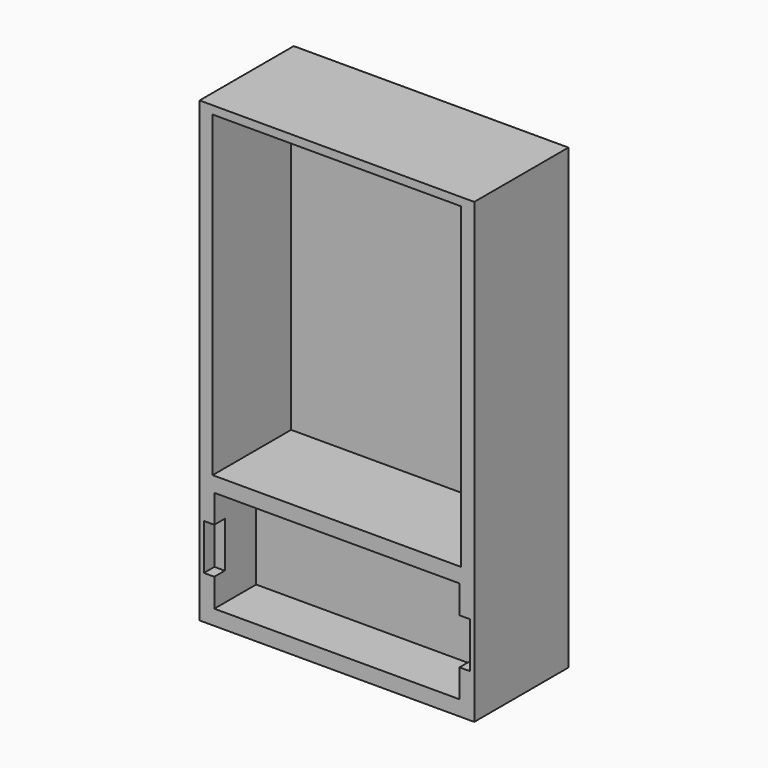
from build123d import *

# Parameters (mm, degrees)
F0_W     = 21
F0_H     = 35
F0_W_2   = 19
F0_H_2   = 24.2712582345
F1_DEPTH = 9
F2_DEPTH = 1.5
F3_DEPTH = 5
F0_W_3   = 0.7944880121
F0_H_3   = 3.5
F4_DEPTH = 8


# Not quite as in the source:
# - a feature names something its author has since deleted; it is built from what else it names


with BuildPart() as f1:
    # F0 (on Front) → F1 (new body)
    with BuildSketch(Plane.XZ):
        Rectangle(F0_W, F0_H)
        Polygon((-9.3731830162, -10.6923110513), (-9.3731830162, -8.5423110513), (9.3731830162, -8.5423110513), (9.3731830162, -10.6923110513), (10.1676710284, -10.6923110513), (10.1676710284, -14.1923110513), (9.3731830162, -14.1923110513), (9.3731830162, -16.3423110513), (-9.3731830162, -16.3423110513), (-9.3731830162, -14.1923110513), (-10.1676710284, -14.1923110513), (-10.1676710284, -10.6923110513), align=None, mode=Mode.SUBTRACT)
        with Locations((0, 4.7412435117)):
            Rectangle(F0_W_2, F0_H_2, mode=Mode.SUBTRACT)
    extrude(amount=F1_DEPTH)

    # F0 (on Front) → F2 (join)
    with BuildSketch(Plane.XZ):
        with Locations((0, 4.7412435117)):
            Rectangle(F0_W_2, F0_H_2)
    extrude(amount=F2_DEPTH)

    # F0 (on Front) → F3 (join)
    with BuildSketch(Plane.XZ):
        Polygon((9.3731830162, -8.5423110513), (-9.3731830162, -8.5423110513), (-9.3731830162, -10.6923110513), (-9.3731830162, -14.1923110513), (-9.3731830162, -16.3423110513), (9.3731830162, -16.3423110513), (9.3731830162, -14.1923110513), (9.3731830162, -10.6923110513), align=None)
    extrude(amount=F3_DEPTH)

    # F0 (on Front) → F4 (join)
    with BuildSketch(Plane.XZ):
        with Locations((9.7704270223, -12.4423110513)):
            Rectangle(F0_W_3, F0_H_3)
        with Locations((-9.7704270223, -12.4423110513)):
            Rectangle(F0_W_3, F0_H_3)
    extrude(amount=F4_DEPTH)


solid = f1.part
